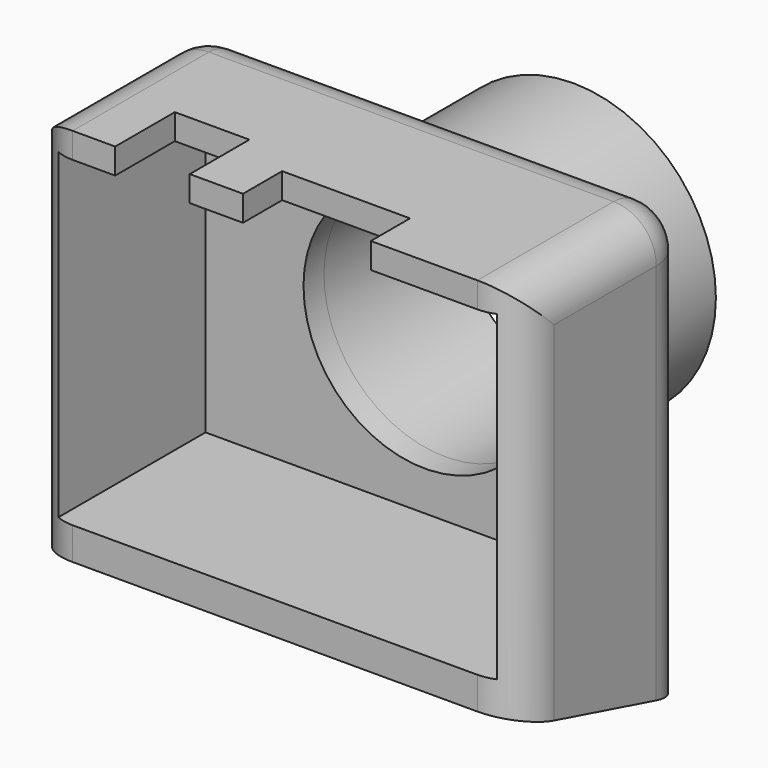
from build123d import *

# Parameters (mm, degrees)
F0_W          = 23
F0_H          = 17.5
F1_DEPTH      = 10
F2_T          = -1.2
F3_R          = 5.7
F4_DEPTH      = 3
F3_R_2        = 6.7
F5_DEPTH      = 7.5
F6_W          = 6
F6_H          = 2.3
F6_W_2        = 3.5
F6_H_2        = 3.5
F7_DEPTH      = 4
F8_DEPTH      = 3
F10_DEPTH     = 30
F11_T1_DEPTH  = 19
F11_T3_DEPTH  = 23.5
F11_T5_DEPTH  = 13
F11_T7_DEPTH  = 27.8205080757
F11_S11_W     = 2
F11_S11_H     = 2
F11_T12_DEPTH = 2
F11_S17_W     = 2
F11_S17_H     = 2
F11_T18_DEPTH = 2


# Not quite as in the source:
# - a fillet or chamfer that OpenCascade refuses, or shapes differently, is made with other operations: its cross-section is extruded or revolved along the edge and cut away or added


with BuildPart() as f1:
    # F0 (on Front) → F1 (new body)
    with BuildSketch(Plane.XZ):
        Rectangle(F0_W, F0_H)
    extrude(amount=F1_DEPTH)

    # F2
    f2_openings = [f1.faces().sort_by_distance(p)[0] for p in [
        (0, -10, 0),
    ]]
    offset(amount=F2_T, openings=f2_openings)

    # F3 (on face) → F4 (cut)
    with BuildSketch(Plane(origin=(0, 0, 0), x_dir=(-1, 0, 0), z_dir=(0, 1, 0))):
        Circle(F3_R)
    extrude(amount=-F4_DEPTH, mode=Mode.SUBTRACT)

    # F3 (on face) → F5 (join)
    with BuildSketch(Plane(origin=(0, 0, 0), x_dir=(-1, 0, 0), z_dir=(0, 1, 0))):
        Circle(F3_R_2)
        Circle(F3_R, mode=Mode.SUBTRACT)
    extrude(amount=F5_DEPTH)

    # F6 (on face) → F7 (cut)
    with BuildSketch(Plane.XY.offset(8.75)):
        with Locations((1.5, -8.85)):
            Rectangle(F6_W, F6_H)
        with Locations((-5.75, -8.25)):
            Rectangle(F6_W_2, F6_H_2)
    extrude(amount=-F7_DEPTH, mode=Mode.SUBTRACT)

    # F8 (add): a face of the model
    f8_faces = [f1.faces().sort_by_distance(p)[0] for p in [
        (0, -5, -8.75),
    ]]
    extrude(f8_faces, amount=F8_DEPTH)

    # F9 (on face) → F10 (cut)
    with BuildSketch(Plane.YZ.offset(11.5)):
        Polygon((-10, -11.75), (0, -11.75), (-10, -9.0705080757), align=None)
    extrude(amount=-F10_DEPTH, mode=Mode.SUBTRACT)

    # F11: fillet of radius 2 on 7 edges, made by hand

    # F11_s2 → F11_t1 (cut)
    with BuildSketch(Plane.YZ.offset(-9.5)):
        with BuildLine():
            ThreePointArc((0, 6.75), (-0.5857864376, 8.1642135624), (-2, 8.75))
            Line((-2, 8.75), (0, 8.75))
            Line((0, 8.75), (0, 6.75))
        make_face()
    extrude(amount=F11_T1_DEPTH, mode=Mode.SUBTRACT)

    # F11_s4 → F11_t3 (cut)
    with BuildSketch(Plane.XY.offset(-16.75)):
        with BuildLine():
            ThreePointArc((-11.5, -2), (-10.9142135624, -0.5857864376), (-9.5, 0))
            Line((-9.5, 0), (-11.5, 0))
            Line((-11.5, 0), (-11.5, -2))
        make_face()
        with BuildLine():
            ThreePointArc((9.5, 0), (10.9142135624, -0.5857864376), (11.5, -2))
            Line((11.5, -2), (11.5, 0))
            Line((11.5, 0), (9.5, 0))
        make_face()
    extrude(amount=F11_T3_DEPTH, mode=Mode.SUBTRACT)

    # F11_s6 → F11_t5 (cut)
    with BuildSketch(Plane.XZ.offset(2)):
        with BuildLine():
            ThreePointArc((9.5, 8.75), (10.9142135624, 8.1642135624), (11.5, 6.75))
            Line((11.5, 6.75), (11.5, 8.75))
            Line((11.5, 8.75), (9.5, 8.75))
        make_face()
        with BuildLine():
            ThreePointArc((-11.5, 6.75), (-10.9142135624, 8.1642135624), (-9.5, 8.75))
            Line((-9.5, 8.75), (-11.5, 8.75))
            Line((-11.5, 8.75), (-11.5, 6.75))
        make_face()
    extrude(amount=F11_T5_DEPTH, mode=Mode.SUBTRACT)

    # F11_s8 → F11_t7 (cut)
    with BuildSketch(Plane.XY.offset(-14.0705080757)):
        with BuildLine():
            ThreePointArc((-11.5, -8), (-10.9142135624, -9.4142135624), (-9.5, -10))
            Line((-9.5, -10), (-11.5, -10))
            Line((-11.5, -10), (-11.5, -8))
        make_face()
        with BuildLine():
            ThreePointArc((9.5, -10), (10.9142135624, -9.4142135624), (11.5, -8))
            Line((11.5, -8), (11.5, -10))
            Line((11.5, -10), (9.5, -10))
        make_face()
    extrude(amount=F11_T7_DEPTH, mode=Mode.SUBTRACT)


with BuildPart() as f11_tool10:
    # F11_s11 → F11_t12 (new body)
    with BuildSketch(Plane.XZ.offset(2)):
        with Locations((10.5, 7.75)):
            Rectangle(F11_S11_W, F11_S11_H)
    extrude(amount=-F11_T12_DEPTH)

    # F11_s13 → F11_t14 (revolve, cut)
    with BuildSketch(Plane(origin=(9.5, -2, 6.75), x_dir=(-0.7071067812, 0, -0.7071067812), z_dir=(0.7071067812, 0, -0.7071067812))):
        with BuildLine():
            ThreePointArc((0, -2), (2, 0), (0, 2))
            Line((0, 2), (0, -2))
        make_face()
    revolve(axis=Axis((9.5, -2, 6.75), (0, 1, 0)), mode=Mode.SUBTRACT)


with BuildPart() as f1_1:
    add(f1.part)

    # F11_t9: cut F11_tool10
    add(f11_tool10.part, mode=Mode.SUBTRACT)


with BuildPart() as f11_tool16:
    # F11_s17 → F11_t18 (new body)
    with BuildSketch(Plane.YZ.offset(-9.5)):
        with Locations((-1, 7.75)):
            Rectangle(F11_S17_W, F11_S17_H)
    extrude(amount=-F11_T18_DEPTH)

    # F11_s19 → F11_t20 (revolve, cut)
    with BuildSketch(Plane(origin=(-9.5, -2, 6.75), x_dir=(0, -0.7071067812, -0.7071067812), z_dir=(0, 0.7071067812, -0.7071067812))):
        with BuildLine():
            ThreePointArc((0, -2), (2, 0), (0, 2))
            Line((0, 2), (0, -2))
        make_face()
    revolve(axis=Axis((-9.5, -2, 6.75), (-1, 0, 0)), mode=Mode.SUBTRACT)


with BuildPart() as f1_2:
    add(f1_1.part)

    # F11_t15: cut F11_tool16
    add(f11_tool16.part, mode=Mode.SUBTRACT)


solid = f1_2.part
